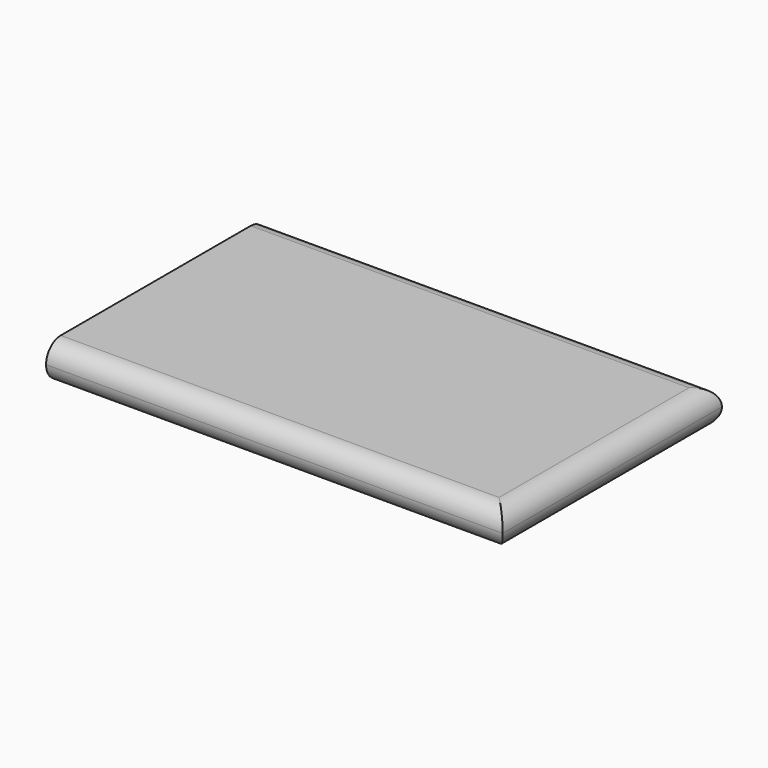
from build123d import *

# Parameters (mm, degrees)
F0_W     = 100
F0_H     = 60
F1_DEPTH = 8
F2_R     = 3.99999


# Not quite as in the source:
# - a fillet or chamfer is up to 0.001 mm smaller than in the source, because OpenCascade refuses the exact size


with BuildPart() as f1:
    # F0 (on Top) → F1 (new body)
    with BuildSketch(Plane.XY):
        Rectangle(F0_W, F0_H)
    extrude(amount=F1_DEPTH)

    # F2 (radius 4 in the source; OpenCascade refuses exactly that, so slightly less here)
    f2_edges = [f1.edges().sort_by_distance(p)[0] for p in [
        (0, -30, 8),
        (0, -30, 0),
        (50, 0, 8),
        (50, 0, 0),
        (0, 30, 8),
        (0, 30, 0),
    ]]
    fillet(f2_edges, radius=F2_R)


solid = f1.part
